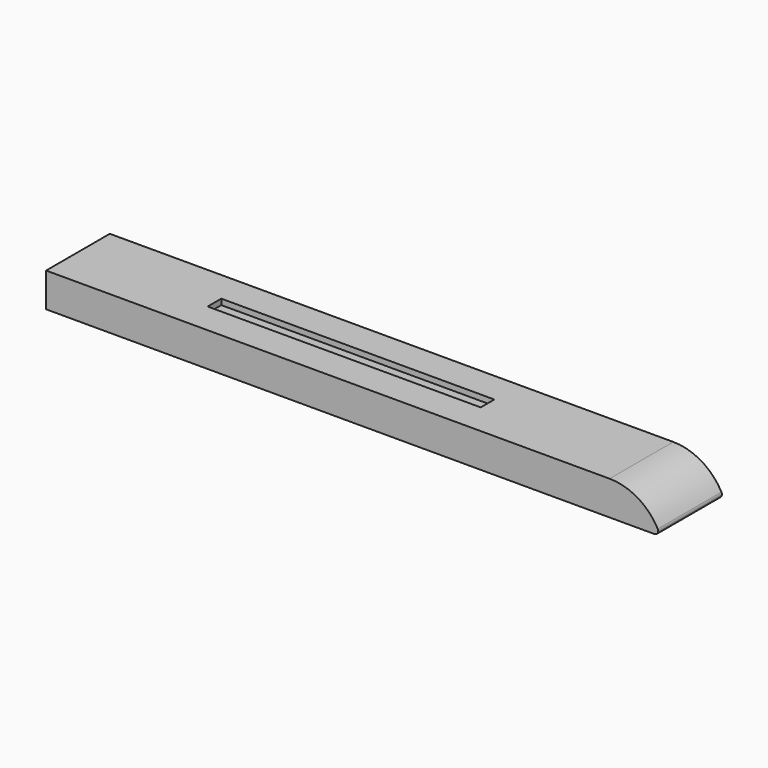
from build123d import *

# Parameters (mm, degrees)
F0_W        = 685.8
F0_H        = 88.9
F0_W_2      = 304.8
F0_H_2      = 19.05
F1_DEPTH    = 38.1
F2_T1_DEPTH = 372.6715659515
F3_R        = 4.2426380505
F4_DEPTH    = 31.75


# Not quite as in the source:
# - a fillet or chamfer that OpenCascade refuses, or shapes differently, is made with other operations: its cross-section is extruded or revolved along the edge and cut away or added


with BuildPart() as f1:
    # F0 (on Top) → F1 (new body)
    with BuildSketch(Plane.XY):
        with Locations((16.0413767457, 5.6168386396)):
            Rectangle(F0_W, F0_H)
        with Locations((-22.0586232543, 5.6168386396)):
            Rectangle(F0_W_2, F0_H_2, mode=Mode.SUBTRACT)
    extrude(amount=F1_DEPTH)

    # F2: fillet of radius 61.3210244843 on 1 edges, made by hand

    # F2_s2 → F2_t1 (cut)
    with BuildSketch(Plane.XZ.offset(-191.9526216153)):
        with BuildLine():
            ThreePointArc((358.9413767457, 0), (336.3654999799, 27.6916706651), (302.1870635554, 38.1))
            Line((302.1870635554, 38.1), (358.9413767457, 38.1))
            Line((358.9413767457, 38.1), (358.9413767457, 0))
        make_face()
    extrude(amount=F2_T1_DEPTH, mode=Mode.SUBTRACT)

    # F3
    f3_edges = [f1.edges().sort_by_distance(p)[0] for p in [
        (358.941377, 5.616839, 0),
    ]]
    fillet(f3_edges, radius=F3_R)

    # F0 (on Top) → F4 (join)
    with BuildSketch(Plane.XY):
        with Locations((-22.0586232543, 5.6168386396)):
            Rectangle(F0_W_2, F0_H_2)
    extrude(amount=F4_DEPTH)


solid = f1.part
